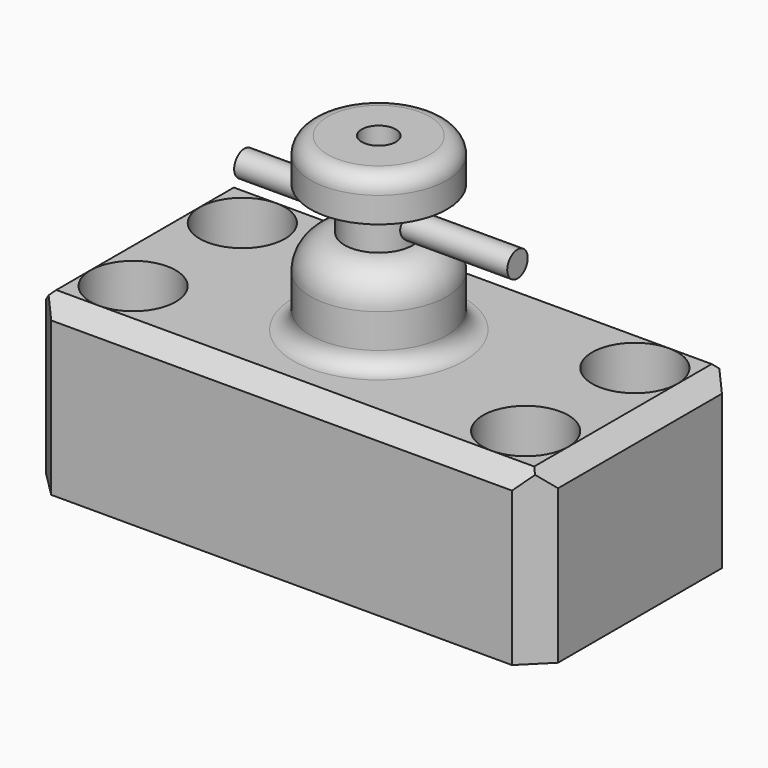
from build123d import *

# Parameters (mm, degrees)
F0_W      = 76.2
F0_H      = 38.1
F1_DEPTH  = 25.4
F2_R      = 6.35
F1_FACE_W = 76.2
F1_FACE_H = 38.1
F3_DEPTH  = 25.4
F4_SIZE   = 2.53999
F5_R      = 10.16
F6_DEPTH  = 38.1
F7_R      = 5.08
F8_DEPTH  = 6.35
F9_R      = 10.16
F10_DEPTH = 6.35
F11_R     = 1.905
F12_DEPTH = 25.4
F13_DEPTH = 15.24
F14_R     = 2.54
F15_R     = 2.54
F16_R     = 2.54
F17_DEPTH = 50.8
F18_SIZE  = 3.81
F19_R     = 5.07999


# Not quite as in the source:
# - a fillet or chamfer is up to 0.001 mm smaller than in the source, because OpenCascade refuses the exact size


with BuildPart() as f1:
    # F0 (on Top) → F1 (new body)
    with BuildSketch(Plane.XY):
        with Locations((-5.318582058, 0.8709464072)):
            Rectangle(F0_W, F0_H)
    extrude(amount=F1_DEPTH)

    # F2 (on Top) + F1_face (on face) → F3 (cut)
    with BuildSketch(Plane.XY):
        with Locations((-34.528582058, -9.2890535928)):
            Circle(F2_R)
        with Locations((23.891417942, 11.0309464072)):
            Circle(F2_R)
        with Locations((23.891417942, -9.2890535928)):
            Circle(F2_R)
        with Locations((-34.528582058, 11.0309464072)):
            Circle(F2_R)
    with BuildSketch(Plane(origin=(-5.318582058, 0.8709464072, 25.4), x_dir=(1, 0, 0), z_dir=(0, 0, 1))):
        Rectangle(F1_FACE_W, F1_FACE_H)
    extrude(amount=F3_DEPTH, mode=Mode.SUBTRACT)

    # F4 (size 2.54 in the source; OpenCascade refuses exactly that, so slightly less here)
    f4_edges = [f1.edges().sort_by_distance(p)[0] for p in [
        (-5.318582, -18.179054, 25.4),
        (32.781418, 0.870946, 25.4),
        (-5.318582, 19.920946, 25.4),
        (-43.418582, 0.870946, 25.4),
    ]]
    chamfer(f4_edges, length=F4_SIZE)

    # F5 (on Top) → F6 (join)
    with BuildSketch(Plane.XY):
        with Locations((-5.3988754862, 0)):
            Circle(F5_R)
    extrude(amount=F6_DEPTH)

    # F7 (on face) → F8 (join)
    with BuildSketch(Plane.XY.offset(38.1)):
        with Locations((-5.3988754862, 0)):
            Circle(F7_R)
    extrude(amount=F8_DEPTH)

    # F9 (on face) → F10 (join)
    with BuildSketch(Plane.XY.offset(44.45)):
        with Locations((-5.3988754862, 0)):
            Circle(F9_R)
    extrude(amount=F10_DEPTH)

    # F11 (on Right) → F12 (join)
    with BuildSketch(Plane.YZ):
        with Locations((0, 40.6930105954)):
            Circle(F11_R)
    extrude(amount=-F12_DEPTH)

    # F11 (on Right) → F13 (join)
    with BuildSketch(Plane.YZ):
        with Locations((0, 40.6930105954)):
            Circle(F11_R)
    extrude(amount=F13_DEPTH)

    # F14
    f14_edges = [f1.edges().sort_by_distance(p)[0] for p in [
        (-15.558875, 0, 25.4),
    ]]
    fillet(f14_edges, radius=F14_R)

    # F15
    f15_edges = [f1.edges().sort_by_distance(p)[0] for p in [
        (-15.558875, 0, 50.8),
    ]]
    fillet(f15_edges, radius=F15_R)

    # F16 (on face) → F17 (cut)
    with BuildSketch(Plane.XY.offset(50.8)):
        with Locations((-5.3988754862, 0)):
            Circle(F16_R)
    extrude(amount=-F17_DEPTH, mode=Mode.SUBTRACT)

    # F18
    f18_edges = [f1.edges().sort_by_distance(p)[0] for p in [
        (32.781418, -18.179054, 11.430005),
        (-43.418582, -18.179054, 11.430005),
        (32.781418, 19.920946, 11.430005),
        (-43.418582, 19.920946, 11.430005),
    ]]
    chamfer(f18_edges, length=F18_SIZE)

    # F19 (radius 5.08 in the source; OpenCascade refuses exactly that, so slightly less here)
    f19_edges = [f1.edges().sort_by_distance(p)[0] for p in [
        (-15.558875, 0, 38.1),
    ]]
    fillet(f19_edges, radius=F19_R)


solid = f1.part
